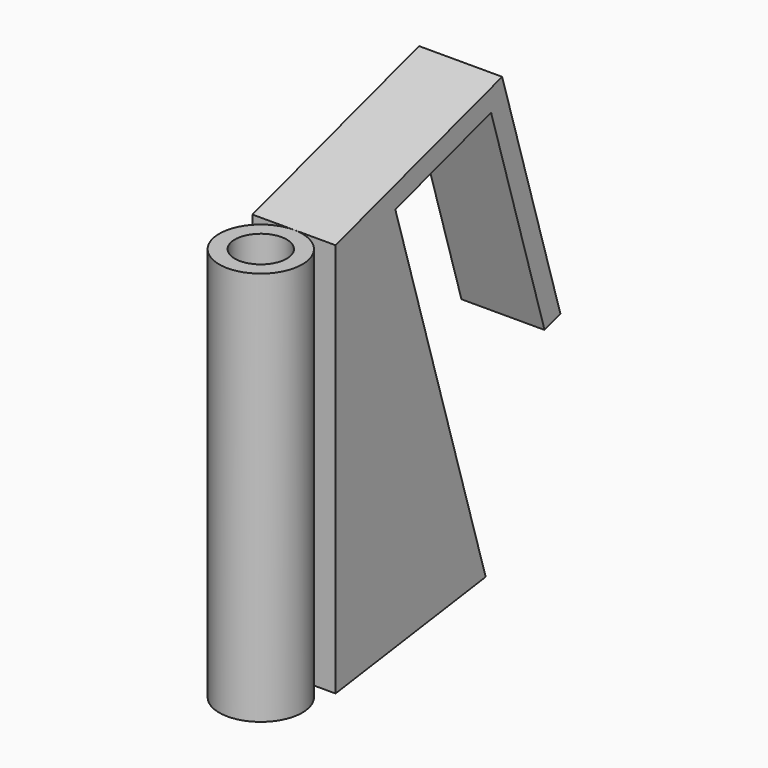
from build123d import *

# Parameters (mm, degrees)
F1_R     = 12.7
F1_R_2   = 7.9375
F2_DEPTH = 120.65
F3_DEPTH = 12.7
F6_DEPTH = 12.7


with BuildPart() as f2:
    # F1 (on Top) → F2 (new body)
    with BuildSketch(Plane.XY):
        with Locations((0, -12.7)):
            Circle(F1_R)
        with Locations((0, -12.7)):
            Circle(F1_R_2, mode=Mode.SUBTRACT)
    extrude(amount=-F2_DEPTH)


with BuildPart() as f3:
    # F0 (on Right) → F3 (new body, symmetric)
    with BuildSketch(Plane.YZ):
        Polygon((97.6843618562, -152.4), (50.8, 0), (0, 0), (0, -152.4), align=None)
        Polygon((0, 0), (50.8, 0), (40.5959168923, 31.3409897747), align=None)
        Polygon((40.5959168923, 31.3409897747), (50.8, 0), (99.3542851518, 14.9372485218), (136.6974064563, -106.4484643576), (185.251691608, -91.5112158358), (165.7442559226, -28.1013051372), (113.4819560317, 57.5799615131), align=None)
    extrude(amount=F3_DEPTH, both=True)


with BuildPart() as f6:
    # F5 (on Right) → F6 (new body, symmetric)
    with BuildSketch(Plane.YZ):
        Polygon((63.6543548718, 19.4610892928), (0, 0), (0, -120.65), (57.3637361695, -112.587100946), (22.8378207674, 0.3420798526), (59.4383799965, 11.5319937674), (79.8605435713, -55.2658934366), (85.9330787717, -53.4093331116), align=None)
    extrude(amount=F6_DEPTH, both=True)


solid = Compound([f2.part, f6.part])
